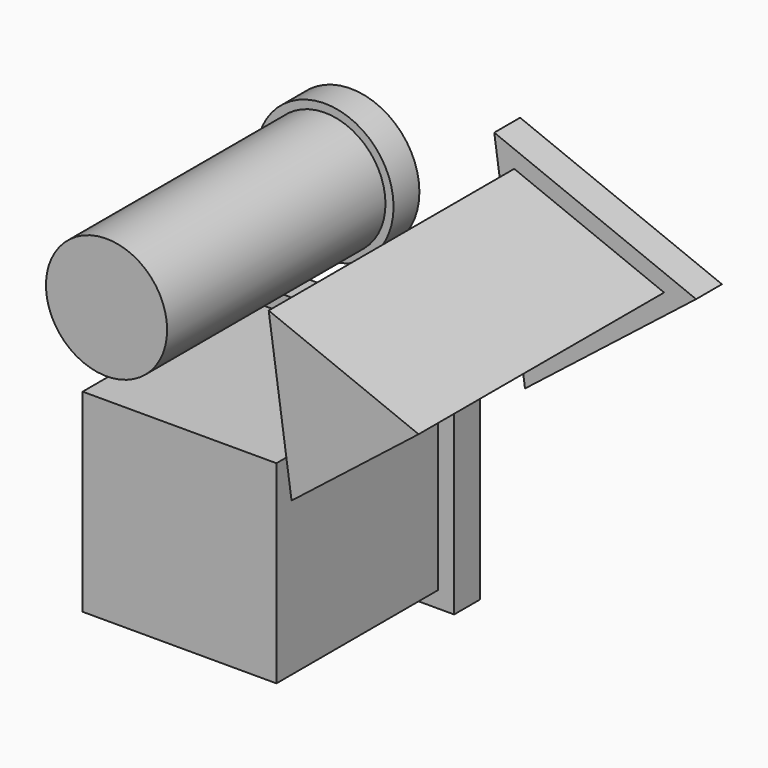
from build123d import *

# Parameters (mm, degrees)
F0_R     = 9.525
F1_DEPTH = 48.006
F0_W     = 30.48
F0_H     = 30.48
F2_DEPTH = 36.83
F3_DEPTH = 53.34
F0_R_2   = 10.795
F4_DEPTH = 5.08
F0_W_2   = 35.56
F0_H_2   = 35.56


# Not quite as in the source:
# - the program builds the solid bodies; features that only make, move or delete a surface that nothing else refers to are left out


with BuildPart() as f1:
    # F0 (on Front) → F1 (new body)
    with BuildSketch(Plane.XZ):
        with Locations((-17.78, 17.78)):
            Circle(F0_R)
    extrude(amount=F1_DEPTH)


with BuildPart() as f2:
    # F0 (on Front) → F2 (new body)
    with BuildSketch(Plane.XZ):
        with Locations((-15.24, -17.78)):
            Rectangle(F0_W, F0_H)
    extrude(amount=F2_DEPTH)


with BuildPart() as f3:
    # F0 (on Front) → F3 (new body)
    with BuildSketch(Plane.XZ):
        Polygon((35.56, 19.7484918216), (11.9879855975, 29.21), (15.5800863581, 4.0652826199), align=None)
    extrude(amount=F3_DEPTH)


with BuildPart() as f4:
    # F0 (on Front) → F4 (new body)
    with BuildSketch(Plane.XZ):
        with Locations((-17.78, 17.78)):
            Circle(F0_R_2)
        with Locations((-17.78, 17.78)):
            Circle(F0_R, mode=Mode.SUBTRACT)
    extrude(amount=F4_DEPTH)


with BuildPart() as f4b:
    # F0 (on Front) → F4, piece 2 (new body)
    with BuildSketch(Plane.XZ):
        with Locations((-15.24, -17.78)):
            Rectangle(F0_W_2, F0_H_2)
        with Locations((-15.24, -17.78)):
            Rectangle(F0_W, F0_H, mode=Mode.SUBTRACT)
    extrude(amount=F4_DEPTH)


with BuildPart() as f4c:
    # F0 (on Front) → F4, piece 3 (new body)
    with BuildSketch(Plane.XZ):
        Polygon((40.588943476, 20.4669119737), (8.8513437572, 33.2059827284), (13.6877847225, -0.6491202606), align=None)
        Polygon((15.5800863581, 4.0652826199), (11.9879855975, 29.21), (35.56, 19.7484918216), align=None, mode=Mode.SUBTRACT)
    extrude(amount=F4_DEPTH)


solid = Compound([f1.part, f2.part, f3.part, f4.part, f4b.part, f4c.part])
